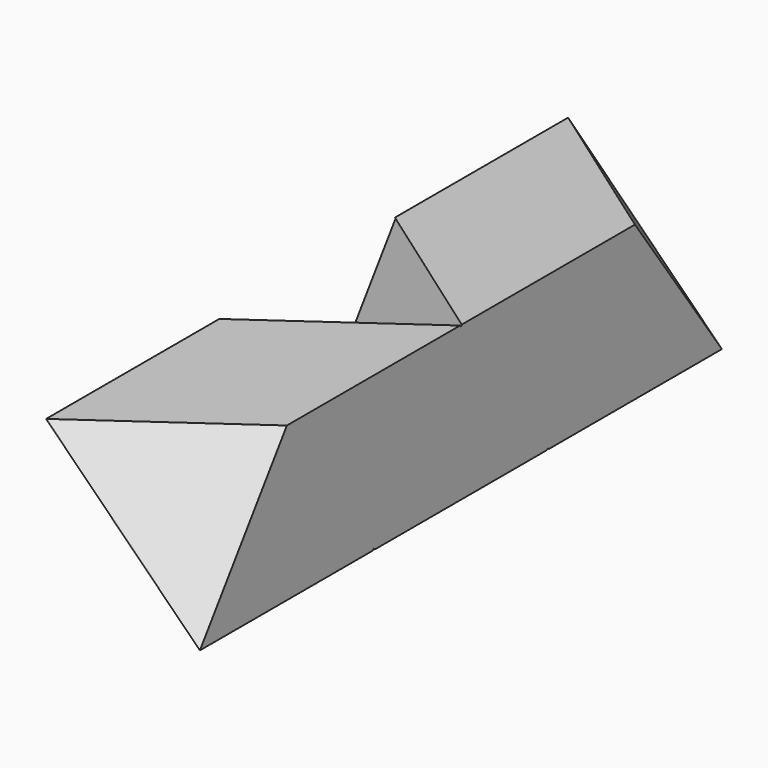
from build123d import *

# Parameters (mm, degrees)
F0_W      = 10.6066017178
F0_H      = 10.6066017178
F1_DEPTH  = 22.5
F4_DEPTH  = 15
F6_DEPTH  = 15
F9_DEPTH  = 15
F11_DEPTH = 15
F13_DEPTH = 15


# Not quite as in the source:
# - a feature names something its author has since deleted; it is built from what else it names


with BuildPart() as f1:
    # F0 (on Front) → F1 (new body, symmetric)
    with BuildSketch(Plane.XZ):
        Rectangle(F0_W, F0_H)
    extrude(amount=F1_DEPTH, both=True)

    # F3 (on 3pt) → F4 (cut, symmetric)
    with BuildSketch(Plane(origin=(0, 0, 0), x_dir=(0, 1, 0), z_dir=(0.7071067812, 0, -0.7071067812))):
        Polygon((-15, -7.5), (-22.5, 0), (-15, 7.5), (-15, 9.5), (-24.5, 9.5), (-24.5, -9.5), (-15, -9.5), align=None)
        Polygon((15, 7.5), (22.5, 0), (15, -7.5), (15, -9.5), (24.5, -9.5), (24.5, 9.5), (15, 9.5), align=None)
    extrude(amount=F4_DEPTH, both=True, mode=Mode.SUBTRACT)

    # F5 (on 3pt) → F6 (cut, symmetric)
    with BuildSketch(Plane(origin=(0, 0, 0), x_dir=(0, 1, 0), z_dir=(0.7071067812, 0, -0.7071067812))):
        Polygon((7.5, 0), (0, -7.5), (-7.5, 0), (-15, -7.5), (-15, -9.5), (15, -9.5), (15, -7.5), align=None)
    extrude(amount=F6_DEPTH, both=True, mode=Mode.SUBTRACT)

    # F8 (on 3pt) → F9 (cut, symmetric)
    with BuildSketch(Plane(origin=(0, 0, 0), x_dir=(0, -1, 0), z_dir=(-0.7071067812, 0, -0.7071067812))):
        Polygon((-7.5, 7.5), (0, 0), (7.5, 7.5), (7.5, 9.5), (-7.5, 9.5), align=None)
    extrude(amount=F9_DEPTH, both=True, mode=Mode.SUBTRACT)

    # F10 (on 3pt) → F11 (cut, symmetric)
    with BuildSketch(Plane(origin=(0, 0, 0), x_dir=(0, 1, 0), z_dir=(0.7071067812, 0, -0.7071067812))):
        Polygon((-17.0707106781, -9.5), (17.0707106781, -9.5), (7.5, 0.0707106781), (0, -7.4292893219), (-7.5, 0.0707106781), align=None)
    extrude(amount=F11_DEPTH, both=True, mode=Mode.SUBTRACT)

    # F12 (on 3pt) → F13 (cut, symmetric)
    with BuildSketch(Plane(origin=(0, 0, 0), x_dir=(0, -1, 0), z_dir=(-0.7071067812, 0, -0.7071067812))):
        Polygon((9.5707106781, 9.5), (-9.5707106781, 9.5), (0, -0.0707106781), align=None)
    extrude(amount=F13_DEPTH, both=True, mode=Mode.SUBTRACT)


solid = f1.part
